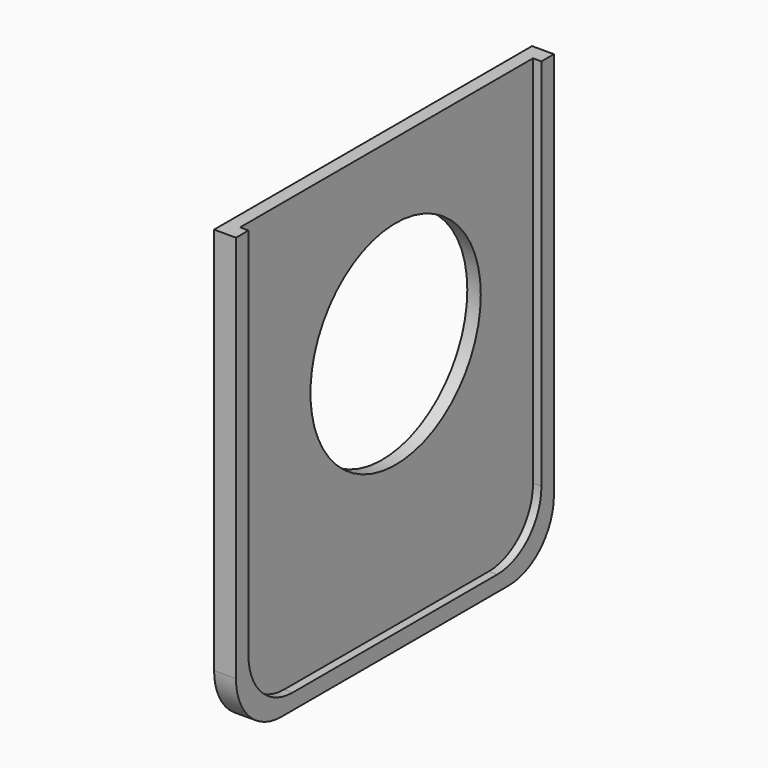
from build123d import *

# Parameters (mm, degrees)
F1_DEPTH  = 7.5
F2_W      = 2.6
F2_H      = 4.75
F0_R      = 18.75
F4_DEPTH  = 2.375
F8_R      = 4
F9_W      = 29.1621480137
F9_H      = 87.7830125391
F9_W_2    = 6.8209778983
F10_DEPTH = 60.1


# Not quite as in the source:
# - a feature names something its author has since deleted; it is built from what else it names


with BuildPart() as f1:
    # F0 (on Right) → F1 (new body)
    with BuildSketch(Plane.YZ):
        with BuildLine():
            Line((-27.5, -30.8578620553), (-27.5, 35))
            Line((-27.5, 35), (-35, 35))
            Line((-35, 35), (-35, -33.3578620553))
            ThreePointArc((-35, -33.3578620553), (-32.0710678119, -40.4289298672), (-25, -43.3578620553))
            Line((-25, -43.3578620553), (25, -43.3578620553))
            ThreePointArc((25, -43.3578620553), (32.0710678119, -40.4289298672), (35, -33.3578620553))
            Line((35, -33.3578620553), (35, 35))
            Line((35, 35), (27.5, 35))
            Line((27.5, 35), (27.5, -30.8578620553))
            ThreePointArc((27.5, -30.8578620553), (26.0355339059, -34.3933959612), (22.5, -35.8578620553))
            Line((22.5, -35.8578620553), (-22.5, -35.8578620553))
            ThreePointArc((-22.5, -35.8578620553), (-26.0355339059, -34.3933959612), (-27.5, -30.8578620553))
        make_face()
    extrude(amount=F1_DEPTH)

    # F3: sweep along a path in F0
    with BuildLine(Plane.YZ) as f3_path:
        Line((27.5, 35), (27.5, -30.8578620553))
        ThreePointArc((27.5, -30.8578620553), (26.0355339059, -34.3933959612), (22.5, -35.8578620553))
        Line((22.5, -35.8578620553), (-22.5, -35.8578620553))
        ThreePointArc((-22.5, -35.8578620553), (-26.0355339059, -34.3933959612), (-27.5, -30.8578620553))
        Line((-27.5, -30.8578620553), (-27.5, 35))
    # F2 (on face) → F3 (sweep, cut)
    with BuildSketch(Plane.XY.offset(35)):
        with Locations((3.675, 29.875)):
            Rectangle(F2_W, F2_H)
    sweep(path=f3_path.line, mode=Mode.SUBTRACT)

    # F0 (on Right) → F4 (join)
    with BuildSketch(Plane.YZ):
        with BuildLine():
            Line((27.5, 35), (-27.5, 35))
            Line((-27.5, 35), (-27.5, -30.8578620553))
            ThreePointArc((-27.5, -30.8578620553), (-26.0355339059, -34.3933959612), (-22.5, -35.8578620553))
            Line((-22.5, -35.8578620553), (22.5, -35.8578620553))
            ThreePointArc((22.5, -35.8578620553), (26.0355339059, -34.3933959612), (27.5, -30.8578620553))
            Line((27.5, -30.8578620553), (27.5, 35))
        make_face()
        with Locations((2, 3)):
            Circle(F0_R, mode=Mode.SUBTRACT)
    extrude(amount=F4_DEPTH)

    # F6 (on offset) → F7 (revolve)
    with BuildSketch(Plane.XY.offset(1)):
        Polygon((0, 22), (0, 25), (-22.6, 35), (-22.6, 32), align=None)
    revolve(axis=Axis((0, 2, 3), (1, 0, 0)))

    # F8
    f8_edges = [f1.edges().sort_by_distance(p)[0] for p in [
        (6.2375, -27.5, 35),
        (6.2375, 27.5, 35),
    ]]
    fillet(f8_edges, radius=F8_R)

    # F9 (on offset) → F10 (cut, symmetric)
    with BuildSketch(Plane.XY.offset(1)):
        with Locations((-14.5810740069, 1.1862572283)):
            Rectangle(F9_W, F9_H)
        with Locations((7.2658261051, 1.1862572283)):
            Rectangle(F9_W_2, F9_H)
    extrude(amount=F10_DEPTH, both=True, mode=Mode.SUBTRACT)


solid = f1.part
